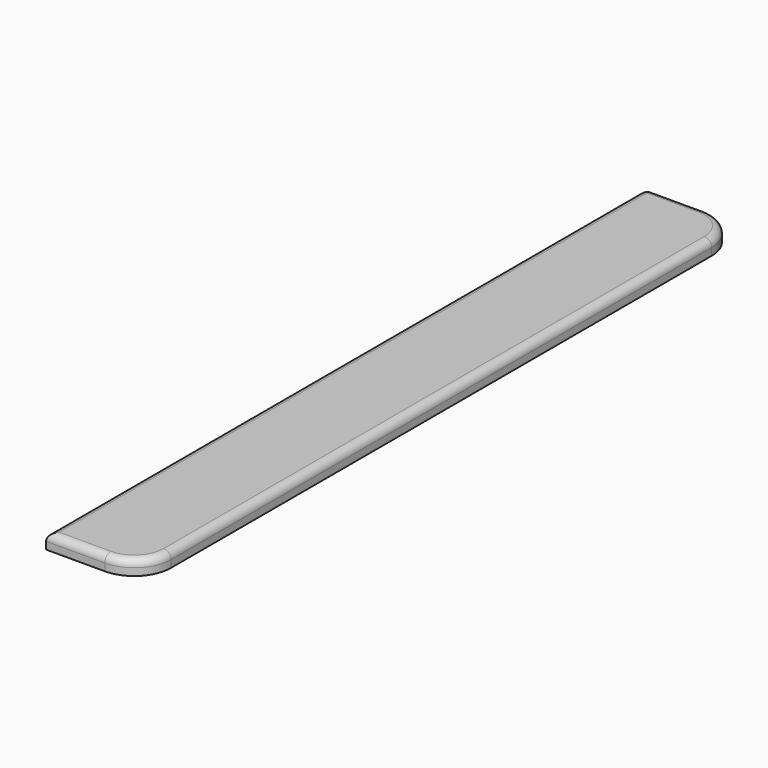
from build123d import *

# Parameters (mm, degrees)
F1_DEPTH     = 2
F2_W         = 1.7
F2_H         = 2
F2_W_2       = 6.3
F2_H_2       = 8
F3_DEPTH     = 1.3
F4_W         = 8
F4_H         = 10
F5_DEPTH     = 2
F6_R         = 5
F7_R         = 1
F8_T1_DEPTH  = 3.3
F8_T3_DEPTH  = 7.5
F8_T5_DEPTH  = 9.5
F8_T7_DEPTH  = 5.5
F8_T9_DEPTH  = 11.5
F8_S13_W     = 1
F8_S13_H     = 1
F8_T14_DEPTH = 1
F8_S19_W     = 1
F8_S19_H     = 1
F8_T20_DEPTH = 1
F8_T24_ANGLE = 90
F10_DEPTH    = 1.3


# Not quite as in the source:
# - a fillet or chamfer that OpenCascade refuses, or shapes differently, is made with other operations: its cross-section is extruded or revolved along the edge and cut away or added


with BuildPart() as f1:
    # F0 (on Top) → F1 (new body)
    with BuildSketch(Plane.XY):
        with BuildLine():
            Line((-6.5, -51), (6.5, -51))
            Line((6.5, -51), (6.5, 46))
            ThreePointArc((6.5, 46), (5.0355339059, 49.5355339059), (1.5, 51))
            Line((1.5, 51), (-6.5, 51))
            Line((-6.5, 51), (-6.5, -51))
        make_face()
    extrude(amount=F1_DEPTH)

    # F2 (on face) → F3 (join)
    with BuildSketch(Plane(origin=(0, 0, 0), x_dir=(1, 0, 0), z_dir=(0, 0, -1))):
        with Locations((-5.65, -50)):
            Rectangle(F2_W, F2_H)
        with Locations((-1.65, -50)):
            Rectangle(F2_W_2, F2_H)
        with Locations((-5.65, -45)):
            Rectangle(F2_W, F2_H_2)
    extrude(amount=F3_DEPTH)

    # F4 (on face) → F5 (join)
    with BuildSketch(Plane(origin=(0, 0, -1.3), x_dir=(1, 0, 0), z_dir=(0, 0, -1))):
        with Locations((-2.5, -46)):
            Rectangle(F4_W, F4_H)
    extrude(amount=F5_DEPTH)

    # F6
    f6_edges = [f1.edges().sort_by_distance(p)[0] for p in [
        (6.5, -51, 1),
        (1.5, 41, -2.3),
    ]]
    fillet(f6_edges, radius=F6_R)

    # F7
    f7_edges = [f1.edges().sort_by_distance(p)[0] for p in [
        (-2.5, -51, 2),
        (5.035534, -49.535534, 2),
        (-6.5, 0, 2),
        (6.5, 0, 2),
        (-2.5, 51, 2),
        (5.035534, 49.535534, 2),
    ]]
    fillet(f7_edges, radius=F7_R)

    # F8: fillet of radius 1 on 6 edges, made by hand

    # F8_s2 → F8_t1 (cut)
    with BuildSketch(Plane.XY.offset(-2.3)):
        with BuildLine():
            ThreePointArc((-5.5, 51), (-6.2071067812, 50.7071067812), (-6.5, 50))
            Line((-6.5, 50), (-6.5, 51))
            Line((-6.5, 51), (-5.5, 51))
        make_face()
    extrude(amount=F8_T1_DEPTH, mode=Mode.SUBTRACT)

    # F8_s4 → F8_t3 (cut)
    with BuildSketch(Plane.XZ.offset(-53.5)):
        with BuildLine():
            ThreePointArc((1.5, -2.3), (1.2071067812, -3.0071067812), (0.5, -3.3))
            Line((0.5, -3.3), (1.5, -3.3))
            Line((1.5, -3.3), (1.5, -2.3))
        make_face()
    extrude(amount=F8_T3_DEPTH, mode=Mode.SUBTRACT)

    # F8_s6 → F8_t5 (cut)
    with BuildSketch(Plane.YZ.offset(-5.5)):
        with BuildLine():
            ThreePointArc((51, -2.3), (50.7071067812, -3.0071067812), (50, -3.3))
            Line((50, -3.3), (51, -3.3))
            Line((51, -3.3), (51, -2.3))
        make_face()
    extrude(amount=F8_T5_DEPTH, mode=Mode.SUBTRACT)

    # F8_s8 → F8_t7 (cut)
    with BuildSketch(Plane.YZ.offset(-9)):
        with BuildLine():
            ThreePointArc((42, -3.3), (41.2928932188, -3.0071067812), (41, -2.3))
            Line((41, -2.3), (41, -3.3))
            Line((41, -3.3), (42, -3.3))
        make_face()
    extrude(amount=F8_T7_DEPTH, mode=Mode.SUBTRACT)

    # F8_s10 → F8_t9 (cut)
    with BuildSketch(Plane.XZ.offset(-50)):
        with BuildLine():
            ThreePointArc((-6.5, -2.3), (-6.2071067812, -3.0071067812), (-5.5, -3.3))
            Line((-5.5, -3.3), (-6.5, -3.3))
            Line((-6.5, -3.3), (-6.5, -2.3))
        make_face()
    extrude(amount=F8_T9_DEPTH, mode=Mode.SUBTRACT)


with BuildPart() as f8_tool12:
    # F8_s13 → F8_t14 (new body)
    with BuildSketch(Plane.XZ.offset(-50)):
        with Locations((-6, 1.5)):
            Rectangle(F8_S13_W, F8_S13_H)
    extrude(amount=-F8_T14_DEPTH)

    # F8_s15 → F8_t16 (revolve, cut)
    with BuildSketch(Plane(origin=(-5.5, 50, 1), x_dir=(0.7071067812, 0, -0.7071067812), z_dir=(0.7071067812, 0, 0.7071067812))):
        with BuildLine():
            ThreePointArc((0, -1), (1, 0), (0, 1))
            Line((0, 1), (0, -1))
        make_face()
    revolve(axis=Axis((-5.5, 50, 1), (0, 1, 0)), mode=Mode.SUBTRACT)


with BuildPart() as f1_1:
    add(f1.part)

    # F8_t11: cut F8_tool12
    add(f8_tool12.part, mode=Mode.SUBTRACT)


with BuildPart() as f8_tool18:
    # F8_s19 → F8_t20 (new body)
    with BuildSketch(Plane.XZ.offset(-50)):
        with Locations((-6, -2.8)):
            Rectangle(F8_S19_W, F8_S19_H)
    extrude(amount=-F8_T20_DEPTH)

    # F8_s21 → F8_t22 (revolve, cut)
    with BuildSketch(Plane(origin=(-5.5, 50, -2.3), x_dir=(0.7071067812, 0, 0.7071067812), z_dir=(-0.7071067812, 0, 0.7071067812))):
        with BuildLine():
            ThreePointArc((0, -1), (1, 0), (0, 1))
            Line((0, 1), (0, -1))
        make_face()
    revolve(axis=Axis((-5.5, 50, -2.3), (0, 1, 0)), mode=Mode.SUBTRACT)


with BuildPart() as f1_2:
    add(f1_1.part)

    # F8_t17: cut F8_tool18
    add(f8_tool18.part, mode=Mode.SUBTRACT)

    # F8_s23 → F8_t24 (revolve, cut)
    with BuildSketch(Plane.XZ.offset(-46)):
        with BuildLine():
            ThreePointArc((0.5, -3.3), (1.2071067812, -3.0071067812), (1.5, -2.3))
            Line((1.5, -2.3), (1.5, -3.3))
            Line((1.5, -3.3), (0.5, -3.3))
        make_face()
    revolve(axis=Axis((-3.5, 46, -3.3), (0, 0, -1)), revolution_arc=F8_T24_ANGLE, mode=Mode.SUBTRACT)

    # F9 (on face) → F10 (join, through all)
    with BuildSketch(Plane(origin=(0, 0, 0), x_dir=(1, 0, 0), z_dir=(0, 0, -1))):
        with BuildLine():
            ThreePointArc((-3.5, -42), (-0.6715728753, -43.1715728753), (0.5, -46))
            Line((0.5, -46), (1.5, -46))
            ThreePointArc((1.5, -46), (0.0355339059, -42.4644660941), (-3.5, -41))
            Line((-3.5, -41), (-3.5, -42))
        make_face()
    extrude(amount=F10_DEPTH)


solid = f1_2.part
